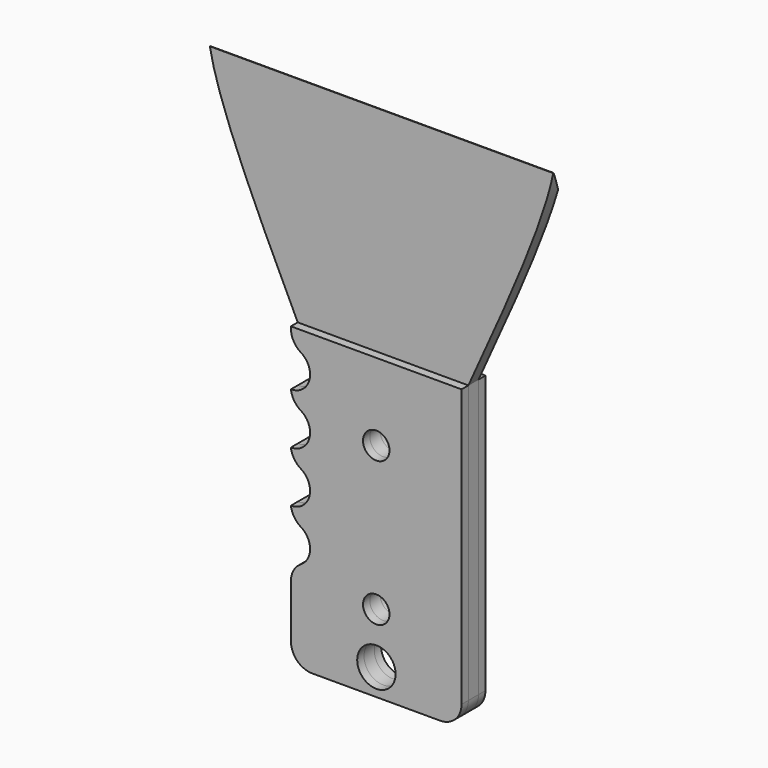
from build123d import *

# Parameters (mm, degrees)
F0_W           = 40
F0_H           = 70
F1_DEPTH       = 3
F2_SIZE2       = 2.8867513459
F2_SIZE        = 5
F3_R           = 5
F5_DEPTH       = 2
F7_DEPTH       = 2
F9_DEPTH       = 25
F10_T1_DEPTH   = 20.8887360535
F10_T3_DEPTH   = 18
F10_2_T1_DEPTH = 19.8887360535
F10_2_T3_DEPTH = 17
F10_3_T1_DEPTH = 19.8887360535
F10_3_T3_DEPTH = 17
F11_R          = 3.1
F12_DEPTH      = 25
F13_R          = 4.5
F14_DEPTH      = 25


# Not quite as in the source:
# - a fillet or chamfer that OpenCascade refuses, or shapes differently, is made with other operations: its cross-section is extruded or revolved along the edge and cut away or added


with BuildPart() as f1:
    # F0 (on Front) → F1 (new body)
    with BuildSketch(Plane.XZ):
        with Locations((-17.71930933, -30.67235291)):
            Rectangle(F0_W, F0_H)
        with BuildLine():
            add(Edge.make_bspline(
                [(-37.71930933, 4.32764709), (-46.9567519014, 23.5397209268), (-56.1941944728, 42.7517947636), (-58.3224408329, 54.5924380422)],
                knots=[0, 0, 0, 0, 0.660266098, 0.660266098, 0.660266098, 0.660266098], degree=3))
            Line((-37.71930933, 4.32764709), (2.28069067, 4.32764709))
            add(Edge.make_bspline(
                [(2.28069067, 4.32764709), (11.0710881678, 23.6786254545), (19.8614856657, 43.029603819), (22.1735145897, 54.5924380422)],
                knots=[0, 0, 0, 0, 0.6674614582, 0.6674614582, 0.6674614582, 0.6674614582], degree=3))
            Line((22.1735145897, 54.5924380422), (-58.3224408329, 54.5924380422))
        make_face()
    extrude(amount=F1_DEPTH)

    # F2
    f2_edges = [f1.edges().sort_by_distance(p)[0] for p in [
        (-18.074463, 0, 54.592438),
    ]]
    f2_side = f1.faces().sort_by_distance((-17.870768, 0, 2.51511))[0]
    chamfer(f2_edges, length=F2_SIZE, length2=F2_SIZE2, reference=f2_side)

    # F3
    f3_edges = [f1.edges().sort_by_distance(p)[0] for p in [
        (2.280691, -1.5, -65.672353),
        (-37.719309, -1.5, -65.672353),
    ]]
    fillet(f3_edges, radius=F3_R)


with BuildPart() as f5:
    # F4 (on face) → F5 (new body)
    with BuildSketch(Plane.XZ.offset(3)):
        with BuildLine():
            Line((2.28069067, 4.32764709), (-37.71930933, 4.32764709))
            Line((-37.71930933, 4.32764709), (-37.71930933, -60.67235291))
            ThreePointArc((-37.71930933, -60.67235291), (-36.2548432359, -64.207886816), (-32.71930933, -65.67235291))
            Line((-32.71930933, -65.67235291), (-2.71930933, -65.67235291))
            ThreePointArc((-2.71930933, -65.67235291), (0.8162245759, -64.207886816), (2.28069067, -60.67235291))
            Line((2.28069067, -60.67235291), (2.28069067, 4.32764709))
        make_face()
    extrude(amount=F5_DEPTH)


with BuildPart() as f7:
    # F6 (on face) → F7 (new body)
    with BuildSketch(Plane(origin=(0, 0, 0), x_dir=(-1, 0, 0), z_dir=(0, 1, 0))):
        with BuildLine():
            Line((37.71930933, 4.32764709), (-2.28069067, 4.32764709))
            Line((-2.28069067, 4.32764709), (-2.28069067, -60.67235291))
            ThreePointArc((-2.28069067, -60.67235291), (-0.8162245759, -64.207886816), (2.71930933, -65.67235291))
            Line((2.71930933, -65.67235291), (32.71930933, -65.67235291))
            ThreePointArc((32.71930933, -65.67235291), (36.2548432359, -64.207886816), (37.71930933, -60.67235291))
            Line((37.71930933, -60.67235291), (37.71930933, 4.32764709))
        make_face()
    extrude(amount=F7_DEPTH)


with BuildPart() as f9_tool:
    # F8 (on face) → F9 (new body)
    with BuildSketch(Plane.XZ.offset(5)):
        with BuildLine():
            ThreePointArc((-37.71930933, -8.67235291), (-34.5373288146, -7.3543334254), (-33.21930933, -4.17235291))
            ThreePointArc((-33.21930933, -4.17235291), (-34.5373288146, -0.9903723947), (-37.71930933, 0.32764709))
            Line((-37.71930933, 0.32764709), (-37.71930933, -8.67235291))
        make_face()
        with BuildLine():
            ThreePointArc((-33.21930933, -16.17235291), (-34.5373288146, -12.9903723947), (-37.71930933, -11.67235291))
            Line((-37.71930933, -11.67235291), (-37.71930933, -20.67235291))
            ThreePointArc((-37.71930933, -20.67235291), (-34.5373288146, -19.3543334254), (-33.21930933, -16.17235291))
        make_face()
        with BuildLine():
            ThreePointArc((-33.21930933, -28.17235291), (-34.5373288146, -24.9903723947), (-37.71930933, -23.67235291))
            Line((-37.71930933, -23.67235291), (-37.71930933, -32.67235291))
            ThreePointArc((-37.71930933, -32.67235291), (-34.5373288146, -31.3543334254), (-33.21930933, -28.17235291))
        make_face()
        with BuildLine():
            ThreePointArc((-33.21930933, -40.17235291), (-34.5373288146, -36.9903723947), (-37.71930933, -35.67235291))
            Line((-37.71930933, -35.67235291), (-37.71930933, -44.67235291))
            ThreePointArc((-37.71930933, -44.67235291), (-34.5373288146, -43.3543334254), (-33.21930933, -40.17235291))
        make_face()
    extrude(amount=-F9_DEPTH)


with BuildPart() as f1_1:
    add(f1.part)

    # F9: cut by f9_tool
    add(f9_tool.part, mode=Mode.SUBTRACT)

    # F10: fillet of radius 5 on 5 edges, made by hand

    # F10_s2 → F10_t1 (cut)
    with BuildSketch(Plane.XZ.offset(-8.9443680268)):
        with BuildLine():
            ThreePointArc((-35.3508882774, -0.3460515997), (-37.0872547702, 1.4720729837), (-37.71930933, 3.9053943007))
            Line((-37.71930933, 3.9053943007), (-37.71930933, 0.32764709))
            ThreePointArc((-37.71930933, 0.32764709), (-36.4881220771, 0.1559467501), (-35.3508882774, -0.3460515997))
        make_face()
        with BuildLine():
            ThreePointArc((-37.71930933, -48.2501001207), (-37.0872547702, -45.8167788038), (-35.3508882774, -43.9986542204))
            ThreePointArc((-35.3508882774, -43.9986542204), (-36.4881220771, -44.5006525702), (-37.71930933, -44.67235291))
            Line((-37.71930933, -44.67235291), (-37.71930933, -48.2501001207))
        make_face()
    extrude(amount=F10_T1_DEPTH, mode=Mode.SUBTRACT)

    # F10_s4 → F10_t3 (cut)
    with BuildSketch(Plane.XZ.offset(-7.5)):
        with BuildLine():
            ThreePointArc((-35.3680027444, -12.3355108048), (-36.9632021222, -10.7732299606), (-37.71930933, -8.67235291))
            Line((-37.71930933, -8.67235291), (-37.71930933, -11.67235291))
            ThreePointArc((-37.71930933, -11.67235291), (-36.4977917234, -11.8413143814), (-35.3680027444, -12.3355108048))
        make_face()
        with BuildLine():
            ThreePointArc((-35.3680027444, -24.3355108048), (-36.9632021222, -22.7732299606), (-37.71930933, -20.67235291))
            Line((-37.71930933, -20.67235291), (-37.71930933, -23.67235291))
            ThreePointArc((-37.71930933, -23.67235291), (-36.4977917234, -23.8413143814), (-35.3680027444, -24.3355108048))
        make_face()
        with BuildLine():
            ThreePointArc((-35.3680027444, -36.3355108048), (-36.9632021222, -34.7732299606), (-37.71930933, -32.67235291))
            Line((-37.71930933, -32.67235291), (-37.71930933, -35.67235291))
            ThreePointArc((-37.71930933, -35.67235291), (-36.4977917234, -35.8413143814), (-35.3680027444, -36.3355108048))
        make_face()
    extrude(amount=F10_T3_DEPTH, mode=Mode.SUBTRACT)


with BuildPart() as f5_1:
    add(f5.part)

    # F9: cut by f9_tool
    add(f9_tool.part, mode=Mode.SUBTRACT)

    # F10#2: fillet of radius 5 on 5 edges, made by hand

    # F10_2_s2 → F10_2_t1 (cut)
    with BuildSketch(Plane.XZ.offset(-5.9443680268)):
        with BuildLine():
            ThreePointArc((-37.71930933, 3.9053943007), (-37.0872547702, 1.4720729837), (-35.3508882774, -0.3460515997))
            ThreePointArc((-35.3508882774, -0.3460515997), (-36.4881220771, 0.1559467501), (-37.71930933, 0.32764709))
            Line((-37.71930933, 0.32764709), (-37.71930933, 3.9053943007))
        make_face()
        with BuildLine():
            ThreePointArc((-37.71930933, -48.2501001207), (-37.0872547702, -45.8167788038), (-35.3508882774, -43.9986542204))
            ThreePointArc((-35.3508882774, -43.9986542204), (-36.4881220771, -44.5006525702), (-37.71930933, -44.67235291))
            Line((-37.71930933, -44.67235291), (-37.71930933, -48.2501001207))
        make_face()
    extrude(amount=F10_2_T1_DEPTH, mode=Mode.SUBTRACT)

    # F10_2_s4 → F10_2_t3 (cut)
    with BuildSketch(Plane.XZ.offset(-4.5)):
        with BuildLine():
            ThreePointArc((-35.3680027444, -12.3355108048), (-36.9632021222, -10.7732299606), (-37.71930933, -8.67235291))
            Line((-37.71930933, -8.67235291), (-37.71930933, -11.67235291))
            ThreePointArc((-37.71930933, -11.67235291), (-36.4977917234, -11.8413143814), (-35.3680027444, -12.3355108048))
        make_face()
        with BuildLine():
            ThreePointArc((-35.3680027444, -24.3355108048), (-36.9632021222, -22.7732299606), (-37.71930933, -20.67235291))
            Line((-37.71930933, -20.67235291), (-37.71930933, -23.67235291))
            ThreePointArc((-37.71930933, -23.67235291), (-36.4977917234, -23.8413143814), (-35.3680027444, -24.3355108048))
        make_face()
        with BuildLine():
            ThreePointArc((-35.3680027444, -36.3355108048), (-36.9632021222, -34.7732299606), (-37.71930933, -32.67235291))
            Line((-37.71930933, -32.67235291), (-37.71930933, -35.67235291))
            ThreePointArc((-37.71930933, -35.67235291), (-36.4977917234, -35.8413143814), (-35.3680027444, -36.3355108048))
        make_face()
    extrude(amount=F10_2_T3_DEPTH, mode=Mode.SUBTRACT)


with BuildPart() as f7_1:
    add(f7.part)

    # F9: cut by f9_tool
    add(f9_tool.part, mode=Mode.SUBTRACT)

    # F10#3: fillet of radius 5 on 5 edges, made by hand

    # F10_3_s2 → F10_3_t1 (cut)
    with BuildSketch(Plane.XZ.offset(-10.9443680268)):
        with BuildLine():
            ThreePointArc((-37.71930933, 3.9053943007), (-37.0872547702, 1.4720729837), (-35.3508882774, -0.3460515997))
            ThreePointArc((-35.3508882774, -0.3460515997), (-36.4881220771, 0.1559467501), (-37.71930933, 0.32764709))
            Line((-37.71930933, 0.32764709), (-37.71930933, 3.9053943007))
        make_face()
        with BuildLine():
            ThreePointArc((-35.3508882774, -43.9986542204), (-37.0872547702, -45.8167788038), (-37.71930933, -48.2501001207))
            Line((-37.71930933, -48.2501001207), (-37.71930933, -44.67235291))
            ThreePointArc((-37.71930933, -44.67235291), (-36.4881220771, -44.5006525702), (-35.3508882774, -43.9986542204))
        make_face()
    extrude(amount=F10_3_T1_DEPTH, mode=Mode.SUBTRACT)

    # F10_3_s4 → F10_3_t3 (cut)
    with BuildSketch(Plane.XZ.offset(-9.5)):
        with BuildLine():
            ThreePointArc((-37.71930933, -8.67235291), (-36.9632021222, -10.7732299606), (-35.3680027444, -12.3355108048))
            ThreePointArc((-35.3680027444, -12.3355108048), (-36.4977917234, -11.8413143814), (-37.71930933, -11.67235291))
            Line((-37.71930933, -11.67235291), (-37.71930933, -8.67235291))
        make_face()
        with BuildLine():
            ThreePointArc((-37.71930933, -20.67235291), (-36.9632021222, -22.7732299606), (-35.3680027444, -24.3355108048))
            ThreePointArc((-35.3680027444, -24.3355108048), (-36.4977917234, -23.8413143814), (-37.71930933, -23.67235291))
            Line((-37.71930933, -23.67235291), (-37.71930933, -20.67235291))
        make_face()
        with BuildLine():
            ThreePointArc((-37.71930933, -32.67235291), (-36.9632021222, -34.7732299606), (-35.3680027444, -36.3355108048))
            ThreePointArc((-35.3680027444, -36.3355108048), (-36.4977917234, -35.8413143814), (-37.71930933, -35.67235291))
            Line((-37.71930933, -35.67235291), (-37.71930933, -32.67235291))
        make_face()
    extrude(amount=F10_3_T3_DEPTH, mode=Mode.SUBTRACT)


with BuildPart() as f12_tool:
    # F11 (on face) → F12 (new body)
    with BuildSketch(Plane(origin=(0, 2, 0), x_dir=(-1, 0, 0), z_dir=(0, 1, 0))):
        with Locations((17.71930933, -13.77235291)):
            Circle(F11_R)
        with Locations((17.71930933, -47.57235291)):
            Circle(F11_R)
    extrude(amount=-F12_DEPTH)


with BuildPart() as f1_2:
    add(f1_1.part)

    # F12: cut by f12_tool
    add(f12_tool.part, mode=Mode.SUBTRACT)


with BuildPart() as f5_2:
    add(f5_1.part)

    # F12: cut by f12_tool
    add(f12_tool.part, mode=Mode.SUBTRACT)


with BuildPart() as f7_2:
    add(f7_1.part)

    # F12: cut by f12_tool
    add(f12_tool.part, mode=Mode.SUBTRACT)


with BuildPart() as f14_tool:
    # F13 (on face) → F14 (new body)
    with BuildSketch(Plane(origin=(0, 2, 0), x_dir=(-1, 0, 0), z_dir=(0, 1, 0))):
        with Locations((17.6835853607, -59.4774961946)):
            Circle(F13_R)
    extrude(amount=-F14_DEPTH)


with BuildPart() as f1_3:
    add(f1_2.part)

    # F14: cut by f14_tool
    add(f14_tool.part, mode=Mode.SUBTRACT)


with BuildPart() as f5_3:
    add(f5_2.part)

    # F14: cut by f14_tool
    add(f14_tool.part, mode=Mode.SUBTRACT)


with BuildPart() as f7_3:
    add(f7_2.part)

    # F14: cut by f14_tool
    add(f14_tool.part, mode=Mode.SUBTRACT)


solid = Compound([f1_3.part, f5_3.part, f7_3.part])
